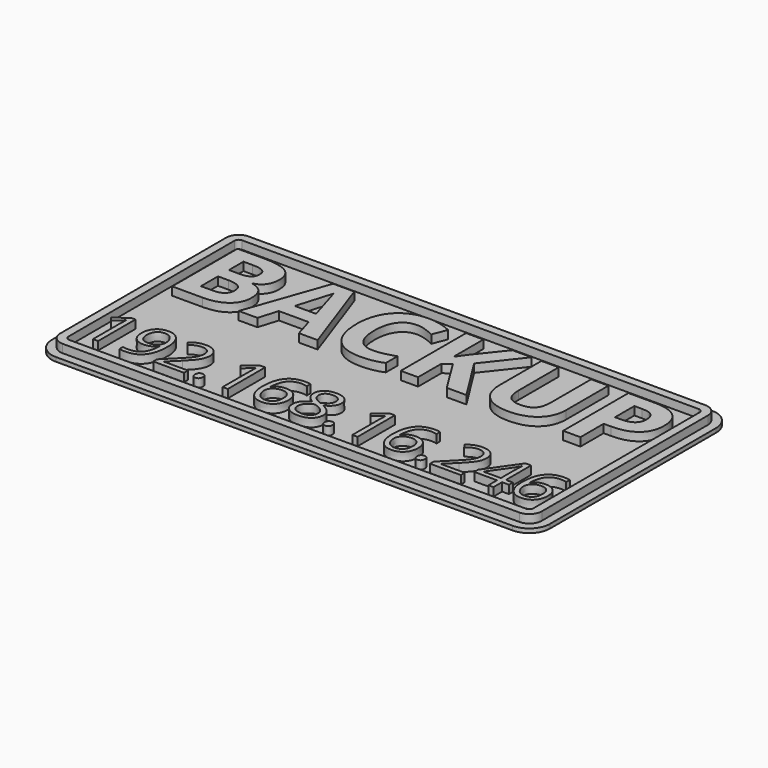
from build123d import *

# Parameters (mm, degrees)
F3_DEPTH       = 1
F4_TEXT_SIZE   = 27.5395727678
F4_TEXT_SIZE_2 = 15.7673610347
F5_DEPTH       = 2


# Not quite as in the source:
# - Text() gives the source's letters only with a copy of the font that has no kerning and outlines rounded to 1/6400 em; it was checked with that copy


with BuildPart() as f3:
    # F2 (on Top) → F3 (new body)
    with BuildSketch(Plane.XY):
        with BuildLine():
            Line((55, 30), (-55, 30))
            ThreePointArc((-55, 30), (-58.5355339059, 28.5355339059), (-60, 25))
            Line((-60, 25), (-60, -25))
            ThreePointArc((-60, -25), (-58.5355339059, -28.5355339059), (-55, -30))
            Line((-55, -30), (55, -30))
            ThreePointArc((55, -30), (58.5355339059, -28.5355339059), (60, -25))
            Line((60, -25), (60, 25))
            ThreePointArc((60, 25), (58.5355339059, 28.5355339059), (55, 30))
        make_face()
    extrude(amount=F3_DEPTH)

    # F4 (on face) → F5 (join)
    with BuildSketch(Plane.XY.offset(1)):
        with BuildLine():
            Line((55, 28), (-55, 28))
            ThreePointArc((-55, 28), (-57.1213203436, 27.1213203436), (-58, 25))
            Line((-58, 25), (-58, -25))
            ThreePointArc((-58, -25), (-57.1213203436, -27.1213203436), (-55, -28))
            Line((-55, -28), (55, -28))
            ThreePointArc((55, -28), (57.1213203436, -27.1213203436), (58, -25))
            Line((58, -25), (58, 25))
            ThreePointArc((58, 25), (57.1213203436, 27.1213203436), (55, 28))
        make_face()
        with BuildLine():
            ThreePointArc((-56, 25), (-55.7071067812, 25.7071067812), (-55, 26))
            Line((-55, 26), (55, 26))
            ThreePointArc((55, 26), (55.7071067812, 25.7071067812), (56, 25))
            Line((56, 25), (56, -25))
            ThreePointArc((56, -25), (55.7071067812, -25.7071067812), (55, -26))
            Line((55, -26), (-55, -26))
            ThreePointArc((-55, -26), (-55.7071067812, -25.7071067812), (-56, -25))
            Line((-56, -25), (-56, 25))
        make_face(mode=Mode.SUBTRACT)
        with Locations((-56, 3.1358720767)):
            Text('BACKUP', F4_TEXT_SIZE, font='Open Sans', font_style=FontStyle.BOLD, text_align=(TextAlign.LEFT, TextAlign.BOTTOM))
        with Locations((-56, -22.9643644695)):
            Text('192.168.16.246', F4_TEXT_SIZE_2, font='Open Sans', text_align=(TextAlign.LEFT, TextAlign.BOTTOM))
    extrude(amount=F5_DEPTH)


solid = f3.part
